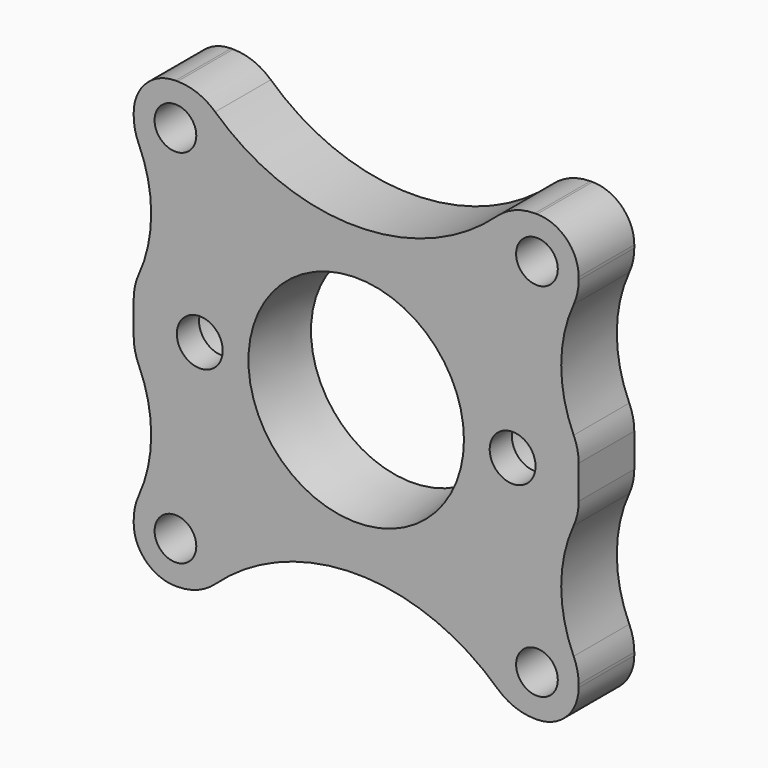
from build123d import *

# Parameters (mm, degrees)
F0_R           = 1.5
F0_R_2         = 7.25
F1_DEPTH       = 5
F2_R           = 3
F3_SIZE2       = 4.99999
F3_SIZE        = 0.49999
F4_D           = 3.3
F4_CBORE_D     = 6.5
F4_CBORE_DEPTH = 3
F5_R           = 4


# Not quite as in the source:
# - a fillet or chamfer is up to 0.001 mm smaller than in the source, because OpenCascade refuses the exact size


with BuildPart() as f1:
    # F0 (on Front) → F1 (new body)
    with BuildSketch(Plane.XZ):
        with BuildLine():
            Line((11.1803398875, -16), (16, -16))
            Line((16, -16), (16, -11.8509778157))
            ThreePointArc((16, -11.8509778157), (14.7445991464, -7), (16, -2.1490221843))
            Line((16, -2.1490221843), (16, 2.1490221843))
            ThreePointArc((16, 2.1490221843), (14.7445991464, 7), (16, 11.8509778157))
            Line((16, 11.8509778157), (16, 16))
            Line((16, 16), (11.1803398875, 16))
            ThreePointArc((11.1803398875, 16), (0, 11), (-11.1803398875, 16))
            Line((-11.1803398875, 16), (-16, 16))
            Line((-16, 16), (-16, 11.8509778157))
            ThreePointArc((-16, 11.8509778157), (-14.7445991464, 7), (-16, 2.1490221843))
            Line((-16, 2.1490221843), (-16, -2.1490221843))
            ThreePointArc((-16, -2.1490221843), (-14.7445991464, -7), (-16, -11.8509778157))
            Line((-16, -11.8509778157), (-16, -16))
            Line((-16, -16), (-11.1803398875, -16))
            ThreePointArc((-11.1803398875, -16), (0, -11), (11.1803398875, -16))
        make_face()
        with Locations((-13, -13)):
            Circle(F0_R, mode=Mode.SUBTRACT)
        with Locations((13, -13)):
            Circle(F0_R, mode=Mode.SUBTRACT)
        with Locations((-13, 13)):
            Circle(F0_R, mode=Mode.SUBTRACT)
        Circle(F0_R_2, mode=Mode.SUBTRACT)
        with Locations((13, 13)):
            Circle(F0_R, mode=Mode.SUBTRACT)
    extrude(amount=F1_DEPTH)

    # F2
    f2_edges = [f1.edges().sort_by_distance(p)[0] for p in [
        (-16, -2.5, 16),
        (16, -2.5, 16),
        (16, -2.5, -16),
        (-16, -2.5, -16),
    ]]
    fillet(f2_edges, radius=F2_R)

    # F3 (size 0.5 and 5 in the source; OpenCascade refuses exactly that, so slightly less here)
    f3_edges = [f1.edges().sort_by_distance(p)[0] for p in [
        (-7.25, -5, 0),
    ]]
    f3_side = f1.faces().sort_by_distance((-15.547452, -5, -12.425489))[0]
    chamfer(f3_edges, length=F3_SIZE, length2=F3_SIZE2, reference=f3_side)

    # F4 (through all)
    with Locations(Plane(origin=(0, 0, 0), x_dir=(1, 0, 0), z_dir=(0, 1, 0))):
        with Locations((11.25, 0), (-11.25, 0)):
            CounterBoreHole(F4_D / 2, F4_CBORE_D / 2, F4_CBORE_DEPTH)

    # F5
    f5_edges = [f1.edges().sort_by_distance(p)[0] for p in [
        (-16, -2.5, -2.149022),
        (-16, -2.5, 2.149022),
        (-16, -2.5, 13),
        (11.18034, -2.5, 16),
        (16, -2.5, 2.149022),
        (16, -2.5, -2.149022),
        (11.18034, -2.5, -16),
        (-16, -2.5, -11.850978),
        (-11.18034, -2.5, -16),
        (-16, -2.5, 11.850978),
        (16, -2.5, -11.850978),
        (-11.18034, -2.5, 16),
        (16, -2.5, 11.850978),
    ]]
    fillet(f5_edges, radius=F5_R)


solid = f1.part
